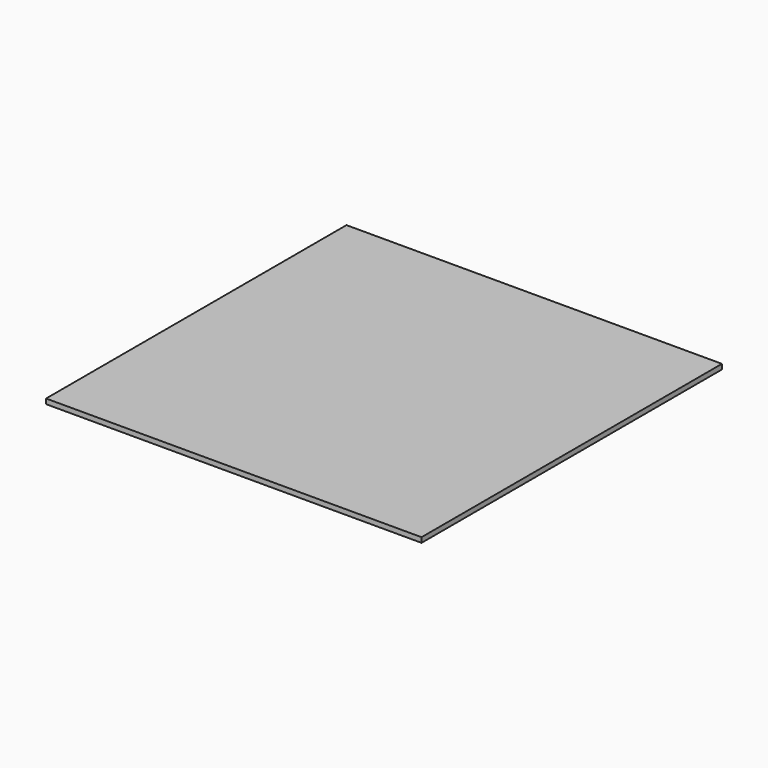
from build123d import *

# Parameters (mm, degrees)
F0_W     = 150
F0_H     = 150
F1_DEPTH = 2


# Not quite as in the source:
# - a feature of the source that left no trace in its solid (it failed there, or was rolled back) is left out


with BuildPart() as f1:
    # F0 (on Top) → F1 (new body)
    with BuildSketch(Plane.XY):
        Rectangle(F0_W, F0_H)
    extrude(amount=F1_DEPTH)


solid = f1.part
